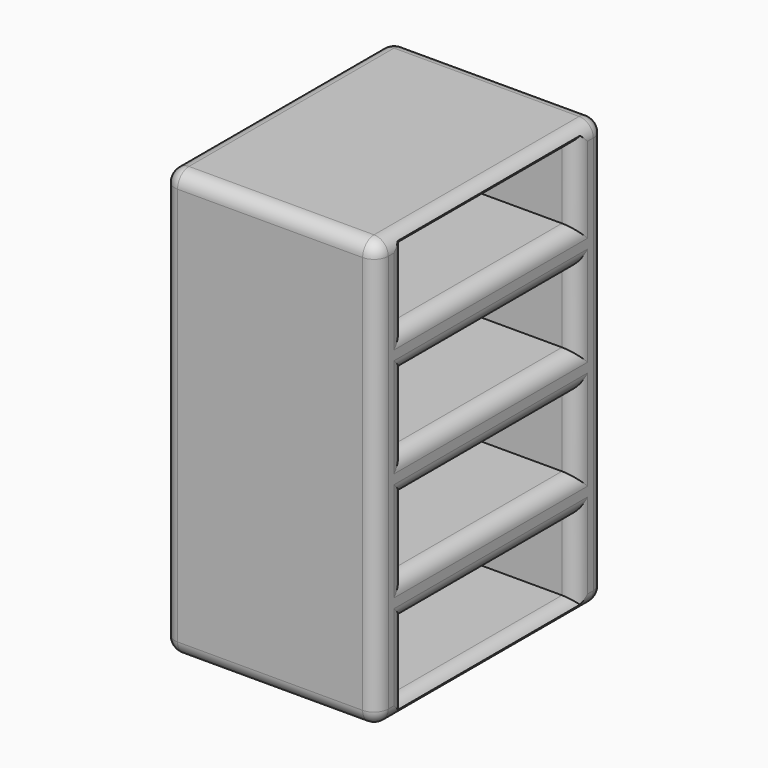
from build123d import *

# Parameters (mm, degrees)
F0_W          = 76.2
F0_H          = 101.6
F1_DEPTH      = 152.4
F2_W          = 76.2
F2_H          = 25.4
F3_DEPTH      = 63.5
F4_T1_DEPTH   = 101.6
F4_T3_DEPTH   = 38.1
F4_T5_DEPTH   = 50.8
F4_T7_DEPTH   = 50.8
F4_T9_DEPTH   = 38.1
F4_T11_DEPTH  = 142.24
F4_T13_DEPTH  = 66.04
F4_T15_DEPTH  = 91.44
F4_T17_DEPTH  = 25.4
F4_T19_DEPTH  = 76.2
F4_T21_DEPTH  = 25.4
F4_T23_DEPTH  = 25.4
F4_T25_DEPTH  = 25.4
F4_S29_W      = 5.1816
F4_S29_H      = 5.1816
F4_T30_DEPTH  = 5.1816
F4_S35_W      = 5.1816
F4_S35_H      = 5.1816
F4_T36_DEPTH  = 5.1816
F4_S41_W      = 5.1816
F4_S41_H      = 5.1816
F4_T42_DEPTH  = 5.1816
F4_S47_W      = 5.1816
F4_S47_H      = 5.1816
F4_T48_DEPTH  = 5.1816
F4_S53_W      = 5.1816
F4_S53_H      = 5.1816
F4_T54_DEPTH  = 5.1816
F4_S59_W      = 5.1816
F4_S59_H      = 5.1816
F4_T60_DEPTH  = 5.1816
F4_S65_W      = 5.1816
F4_S65_H      = 5.1816
F4_T66_DEPTH  = 5.1816
F4_S71_W      = 5.1816
F4_S71_H      = 5.1816
F4_T72_DEPTH  = 5.1816
F4_T79_DEPTH  = 38.1
F4_T84_DEPTH  = 88.9
F4_T91_DEPTH  = 38.1
F4_T95_DEPTH  = 88.9
F4_T102_DEPTH = 88.9
F4_T106_DEPTH = 38.1
F4_T114_DEPTH = 38.1
F4_T118_DEPTH = 88.9
F4_T125_DEPTH = 38.1
F4_T129_DEPTH = 88.9
F4_T136_DEPTH = 38.1
F4_T140_DEPTH = 88.9
F4_T147_DEPTH = 88.9
F4_T151_DEPTH = 38.1
F4_T158_DEPTH = 38.1
F4_T162_DEPTH = 88.9
F4_T169_DEPTH = 38.1
F4_T173_DEPTH = 88.9
F4_T180_DEPTH = 38.1
F4_T184_DEPTH = 88.9
F4_T191_DEPTH = 88.9
F4_T195_DEPTH = 38.1
F4_T202_DEPTH = 38.1
F4_T206_DEPTH = 88.9
F4_T213_DEPTH = 38.1
F4_T217_DEPTH = 88.9
F4_T224_DEPTH = 38.1
F4_T229_DEPTH = 88.9
F4_T236_DEPTH = 88.9
F4_T240_DEPTH = 38.1
F4_T247_DEPTH = 38.1
F4_T252_DEPTH = 88.9


# Not quite as in the source:
# - a fillet or chamfer that OpenCascade refuses, or shapes differently, is made with other operations: its cross-section is extruded or revolved along the edge and cut away or added


with BuildPart() as f1:
    # F0 (on Top) → F1 (new body)
    with BuildSketch(Plane.XY):
        with Locations((2.9496792704, 19.608187279)):
            Rectangle(F0_W, F0_H)
    extrude(amount=F1_DEPTH)

    # F2 (on face) → F3 (cut)
    with BuildSketch(Plane.YZ.offset(41.0496792704)):
        with Locations((19.608187279, 134.62)):
            Rectangle(F2_W, F2_H)
        with Locations((19.608187279, 95.6733333333)):
            Rectangle(F2_W, F2_H)
        with Locations((19.608187279, 56.7266666667)):
            Rectangle(F2_W, F2_H)
        with Locations((19.608187279, 17.78)):
            Rectangle(F2_W, F2_H)
    extrude(amount=-F3_DEPTH, mode=Mode.SUBTRACT)

    # F4: fillet of radius 5.08 on 44 edges, made by hand

    # F4_s2 → F4_t1 (join)
    with BuildSketch(Plane.XZ.offset(-70.408187279)):
        with BuildLine():
            ThreePointArc((-17.3703207296, 121.92), (-20.962423178, 123.4078975516), (-22.4503207296, 127))
            Line((-22.4503207296, 127), (-22.4503207296, 121.92))
            Line((-22.4503207296, 121.92), (-17.3703207296, 121.92))
        make_face()
        with BuildLine():
            ThreePointArc((-17.3703207296, 147.32), (-20.962423178, 145.8321024484), (-22.4503207296, 142.24))
            Line((-22.4503207296, 142.24), (-22.4503207296, 147.32))
            Line((-22.4503207296, 147.32), (-17.3703207296, 147.32))
        make_face()
        with BuildLine():
            ThreePointArc((-17.3703207296, 82.9733333333), (-20.962423178, 84.4612308849), (-22.4503207296, 88.0533333333))
            Line((-22.4503207296, 88.0533333333), (-22.4503207296, 82.9733333333))
            Line((-22.4503207296, 82.9733333333), (-17.3703207296, 82.9733333333))
        make_face()
        with BuildLine():
            ThreePointArc((-17.3703207296, 108.3733333333), (-20.962423178, 106.8854357818), (-22.4503207296, 103.2933333333))
            Line((-22.4503207296, 103.2933333333), (-22.4503207296, 108.3733333333))
            Line((-22.4503207296, 108.3733333333), (-17.3703207296, 108.3733333333))
        make_face()
        with BuildLine():
            ThreePointArc((-17.3703207296, 44.0266666667), (-20.962423178, 45.5145642182), (-22.4503207296, 49.1066666667))
            Line((-22.4503207296, 49.1066666667), (-22.4503207296, 44.0266666667))
            Line((-22.4503207296, 44.0266666667), (-17.3703207296, 44.0266666667))
        make_face()
        with BuildLine():
            ThreePointArc((-17.3703207296, 69.4266666667), (-20.962423178, 67.9387691151), (-22.4503207296, 64.3466666667))
            Line((-22.4503207296, 64.3466666667), (-22.4503207296, 69.4266666667))
            Line((-22.4503207296, 69.4266666667), (-17.3703207296, 69.4266666667))
        make_face()
        with BuildLine():
            ThreePointArc((-17.3703207296, 5.08), (-20.962423178, 6.5678975516), (-22.4503207296, 10.16))
            Line((-22.4503207296, 10.16), (-22.4503207296, 5.08))
            Line((-22.4503207296, 5.08), (-17.3703207296, 5.08))
        make_face()
        with BuildLine():
            ThreePointArc((-17.3703207296, 30.48), (-20.962423178, 28.9921024484), (-22.4503207296, 25.4))
            Line((-22.4503207296, 25.4), (-22.4503207296, 30.48))
            Line((-22.4503207296, 30.48), (-17.3703207296, 30.48))
        make_face()
    extrude(amount=F4_T1_DEPTH)

    # F4_s4 → F4_t3 (join)
    with BuildSketch(Plane.XY.offset(109.22)):
        with BuildLine():
            ThreePointArc((-17.3703207296, 57.708187279), (-20.962423178, 56.2202897274), (-22.4503207296, 52.628187279))
            Line((-22.4503207296, 52.628187279), (-22.4503207296, 57.708187279))
            Line((-22.4503207296, 57.708187279), (-17.3703207296, 57.708187279))
        make_face()
        with BuildLine():
            ThreePointArc((-17.3703207296, -18.491812721), (-20.962423178, -17.0039151694), (-22.4503207296, -13.411812721))
            Line((-22.4503207296, -13.411812721), (-22.4503207296, -18.491812721))
            Line((-22.4503207296, -18.491812721), (-17.3703207296, -18.491812721))
        make_face()
    extrude(amount=F4_T3_DEPTH)

    # F4_s6 → F4_t5 (join)
    with BuildSketch(Plane.XY.offset(70.2733333333)):
        with BuildLine():
            ThreePointArc((-17.3703207296, 57.708187279), (-20.962423178, 56.2202897274), (-22.4503207296, 52.628187279))
            Line((-22.4503207296, 52.628187279), (-22.4503207296, 57.708187279))
            Line((-22.4503207296, 57.708187279), (-17.3703207296, 57.708187279))
        make_face()
        with BuildLine():
            ThreePointArc((-17.3703207296, -18.491812721), (-20.962423178, -17.0039151694), (-22.4503207296, -13.411812721))
            Line((-22.4503207296, -13.411812721), (-22.4503207296, -18.491812721))
            Line((-22.4503207296, -18.491812721), (-17.3703207296, -18.491812721))
        make_face()
    extrude(amount=F4_T5_DEPTH)

    # F4_s8 → F4_t7 (join)
    with BuildSketch(Plane.XY.offset(31.3266666667)):
        with BuildLine():
            ThreePointArc((-17.3703207296, 57.708187279), (-20.962423178, 56.2202897274), (-22.4503207296, 52.628187279))
            Line((-22.4503207296, 52.628187279), (-22.4503207296, 57.708187279))
            Line((-22.4503207296, 57.708187279), (-17.3703207296, 57.708187279))
        make_face()
        with BuildLine():
            ThreePointArc((-17.3703207296, -18.491812721), (-20.962423178, -17.0039151694), (-22.4503207296, -13.411812721))
            Line((-22.4503207296, -13.411812721), (-22.4503207296, -18.491812721))
            Line((-22.4503207296, -18.491812721), (-17.3703207296, -18.491812721))
        make_face()
    extrude(amount=F4_T7_DEPTH)

    # F4_s10 → F4_t9 (join)
    with BuildSketch(Plane.XY.offset(5.08)):
        with BuildLine():
            ThreePointArc((-17.3703207296, 57.708187279), (-20.962423178, 56.2202897274), (-22.4503207296, 52.628187279))
            Line((-22.4503207296, 52.628187279), (-22.4503207296, 57.708187279))
            Line((-22.4503207296, 57.708187279), (-17.3703207296, 57.708187279))
        make_face()
        with BuildLine():
            ThreePointArc((-17.3703207296, -18.491812721), (-20.962423178, -17.0039151694), (-22.4503207296, -13.411812721))
            Line((-22.4503207296, -13.411812721), (-22.4503207296, -18.491812721))
            Line((-22.4503207296, -18.491812721), (-17.3703207296, -18.491812721))
        make_face()
    extrude(amount=F4_T9_DEPTH)

    # F4_s12 → F4_t11 (cut)
    with BuildSketch(Plane.XY.offset(5.08)):
        with BuildLine():
            ThreePointArc((-35.1503207296, -26.111812721), (-33.662423178, -29.7039151694), (-30.0703207296, -31.191812721))
            Line((-30.0703207296, -31.191812721), (-35.1503207296, -31.191812721))
            Line((-35.1503207296, -31.191812721), (-35.1503207296, -26.111812721))
        make_face()
        with BuildLine():
            ThreePointArc((41.0496792704, -26.111812721), (39.5617817188, -29.7039151694), (35.9696792704, -31.191812721))
            Line((35.9696792704, -31.191812721), (41.0496792704, -31.191812721))
            Line((41.0496792704, -31.191812721), (41.0496792704, -26.111812721))
        make_face()
        with BuildLine():
            ThreePointArc((35.9696792704, 70.408187279), (39.5617817188, 68.9202897274), (41.0496792704, 65.328187279))
            Line((41.0496792704, 65.328187279), (41.0496792704, 70.408187279))
            Line((41.0496792704, 70.408187279), (35.9696792704, 70.408187279))
        make_face()
        with BuildLine():
            ThreePointArc((-30.0703207296, 70.408187279), (-33.662423178, 68.9202897274), (-35.1503207296, 65.328187279))
            Line((-35.1503207296, 65.328187279), (-35.1503207296, 70.408187279))
            Line((-35.1503207296, 70.408187279), (-30.0703207296, 70.408187279))
        make_face()
    extrude(amount=F4_T11_DEPTH, mode=Mode.SUBTRACT)

    # F4_s14 → F4_t13 (cut)
    with BuildSketch(Plane.YZ.offset(-30.0703207296)):
        with BuildLine():
            ThreePointArc((-26.111812721, 0), (-29.7039151694, 1.4878975516), (-31.191812721, 5.08))
            Line((-31.191812721, 5.08), (-31.191812721, 0))
            Line((-31.191812721, 0), (-26.111812721, 0))
        make_face()
        with BuildLine():
            ThreePointArc((-26.111812721, 152.4), (-29.7039151694, 150.9121024484), (-31.191812721, 147.32))
            Line((-31.191812721, 147.32), (-31.191812721, 152.4))
            Line((-31.191812721, 152.4), (-26.111812721, 152.4))
        make_face()
        with BuildLine():
            ThreePointArc((70.408187279, 5.08), (68.9202897274, 1.4878975516), (65.328187279, 0))
            Line((65.328187279, 0), (70.408187279, 0))
            Line((70.408187279, 0), (70.408187279, 5.08))
        make_face()
        with BuildLine():
            ThreePointArc((70.408187279, 147.32), (68.9202897274, 150.9121024484), (65.328187279, 152.4))
            Line((65.328187279, 152.4), (70.408187279, 152.4))
            Line((70.408187279, 152.4), (70.408187279, 147.32))
        make_face()
    extrude(amount=F4_T13_DEPTH, mode=Mode.SUBTRACT)

    # F4_s16 → F4_t15 (cut)
    with BuildSketch(Plane.XZ.offset(-65.328187279)):
        with BuildLine():
            ThreePointArc((-30.0703207296, 0), (-33.662423178, 1.4878975516), (-35.1503207296, 5.08))
            Line((-35.1503207296, 5.08), (-35.1503207296, 0))
            Line((-35.1503207296, 0), (-30.0703207296, 0))
        make_face()
        with BuildLine():
            ThreePointArc((41.0496792704, 5.08), (39.5617817188, 1.4878975516), (35.9696792704, 0))
            Line((35.9696792704, 0), (41.0496792704, 0))
            Line((41.0496792704, 0), (41.0496792704, 5.08))
        make_face()
        with BuildLine():
            ThreePointArc((-30.0703207296, 152.4), (-33.662423178, 150.9121024484), (-35.1503207296, 147.32))
            Line((-35.1503207296, 147.32), (-35.1503207296, 152.4))
            Line((-35.1503207296, 152.4), (-30.0703207296, 152.4))
        make_face()
        with BuildLine():
            ThreePointArc((41.0496792704, 147.32), (39.5617817188, 150.9121024484), (35.9696792704, 152.4))
            Line((35.9696792704, 152.4), (41.0496792704, 152.4))
            Line((41.0496792704, 152.4), (41.0496792704, 147.32))
        make_face()
    extrude(amount=F4_T15_DEPTH, mode=Mode.SUBTRACT)

    # F4_s18 → F4_t17 (cut)
    with BuildSketch(Plane.XY.offset(121.92)):
        with BuildLine():
            ThreePointArc((41.0496792704, -23.571812721), (39.5617817188, -19.9797102726), (35.9696792704, -18.491812721))
            Line((35.9696792704, -18.491812721), (41.0496792704, -18.491812721))
            Line((41.0496792704, -18.491812721), (41.0496792704, -23.571812721))
        make_face()
        with BuildLine():
            ThreePointArc((41.0496792704, 62.788187279), (39.5617817188, 59.1960848306), (35.9696792704, 57.708187279))
            Line((35.9696792704, 57.708187279), (41.0496792704, 57.708187279))
            Line((41.0496792704, 57.708187279), (41.0496792704, 62.788187279))
        make_face()
    extrude(amount=F4_T17_DEPTH, mode=Mode.SUBTRACT)

    # F4_s20 → F4_t19 (cut)
    with BuildSketch(Plane.XZ.offset(-57.708187279)):
        with BuildLine():
            ThreePointArc((41.0496792704, 152.4), (39.5617817188, 148.8078975516), (35.9696792704, 147.32))
            Line((35.9696792704, 147.32), (41.0496792704, 147.32))
            Line((41.0496792704, 147.32), (41.0496792704, 152.4))
        make_face()
        with BuildLine():
            ThreePointArc((41.0496792704, 116.84), (39.5617817188, 120.4321024484), (35.9696792704, 121.92))
            Line((35.9696792704, 121.92), (41.0496792704, 121.92))
            Line((41.0496792704, 121.92), (41.0496792704, 116.84))
        make_face()
        with BuildLine():
            ThreePointArc((41.0496792704, 113.4533333333), (39.5617817188, 109.8612308849), (35.9696792704, 108.3733333333))
            Line((35.9696792704, 108.3733333333), (41.0496792704, 108.3733333333))
            Line((41.0496792704, 108.3733333333), (41.0496792704, 113.4533333333))
        make_face()
        with BuildLine():
            ThreePointArc((41.0496792704, 77.8933333333), (39.5617817188, 81.4854357818), (35.9696792704, 82.9733333333))
            Line((35.9696792704, 82.9733333333), (41.0496792704, 82.9733333333))
            Line((41.0496792704, 82.9733333333), (41.0496792704, 77.8933333333))
        make_face()
        with BuildLine():
            ThreePointArc((41.0496792704, 74.5066666667), (39.5617817188, 70.9145642182), (35.9696792704, 69.4266666667))
            Line((35.9696792704, 69.4266666667), (41.0496792704, 69.4266666667))
            Line((41.0496792704, 69.4266666667), (41.0496792704, 74.5066666667))
        make_face()
        with BuildLine():
            ThreePointArc((41.0496792704, 38.9466666667), (39.5617817188, 42.5387691151), (35.9696792704, 44.0266666667))
            Line((35.9696792704, 44.0266666667), (41.0496792704, 44.0266666667))
            Line((41.0496792704, 44.0266666667), (41.0496792704, 38.9466666667))
        make_face()
        with BuildLine():
            ThreePointArc((41.0496792704, 35.56), (39.5617817188, 31.9678975516), (35.9696792704, 30.48))
            Line((35.9696792704, 30.48), (41.0496792704, 30.48))
            Line((41.0496792704, 30.48), (41.0496792704, 35.56))
        make_face()
        with BuildLine():
            ThreePointArc((41.0496792704, 0), (39.5617817188, 3.5921024484), (35.9696792704, 5.08))
            Line((35.9696792704, 5.08), (41.0496792704, 5.08))
            Line((41.0496792704, 5.08), (41.0496792704, 0))
        make_face()
    extrude(amount=F4_T19_DEPTH, mode=Mode.SUBTRACT)

    # F4_s22 → F4_t21 (cut)
    with BuildSketch(Plane.XY.offset(82.9733333333)):
        with BuildLine():
            ThreePointArc((41.0496792704, -23.571812721), (39.5617817188, -19.9797102726), (35.9696792704, -18.491812721))
            Line((35.9696792704, -18.491812721), (41.0496792704, -18.491812721))
            Line((41.0496792704, -18.491812721), (41.0496792704, -23.571812721))
        make_face()
        with BuildLine():
            ThreePointArc((41.0496792704, 62.788187279), (39.5617817188, 59.1960848306), (35.9696792704, 57.708187279))
            Line((35.9696792704, 57.708187279), (41.0496792704, 57.708187279))
            Line((41.0496792704, 57.708187279), (41.0496792704, 62.788187279))
        make_face()
    extrude(amount=F4_T21_DEPTH, mode=Mode.SUBTRACT)

    # F4_s24 → F4_t23 (cut)
    with BuildSketch(Plane.XY.offset(44.0266666667)):
        with BuildLine():
            ThreePointArc((41.0496792704, -23.571812721), (39.5617817188, -19.9797102726), (35.9696792704, -18.491812721))
            Line((35.9696792704, -18.491812721), (41.0496792704, -18.491812721))
            Line((41.0496792704, -18.491812721), (41.0496792704, -23.571812721))
        make_face()
        with BuildLine():
            ThreePointArc((41.0496792704, 62.788187279), (39.5617817188, 59.1960848306), (35.9696792704, 57.708187279))
            Line((35.9696792704, 57.708187279), (41.0496792704, 57.708187279))
            Line((41.0496792704, 57.708187279), (41.0496792704, 62.788187279))
        make_face()
    extrude(amount=F4_T23_DEPTH, mode=Mode.SUBTRACT)

    # F4_s26 → F4_t25 (cut)
    with BuildSketch(Plane.XY.offset(5.08)):
        with BuildLine():
            ThreePointArc((41.0496792704, -23.571812721), (39.5617817188, -19.9797102726), (35.9696792704, -18.491812721))
            Line((35.9696792704, -18.491812721), (41.0496792704, -18.491812721))
            Line((41.0496792704, -18.491812721), (41.0496792704, -23.571812721))
        make_face()
        with BuildLine():
            ThreePointArc((41.0496792704, 62.788187279), (39.5617817188, 59.1960848306), (35.9696792704, 57.708187279))
            Line((35.9696792704, 57.708187279), (41.0496792704, 57.708187279))
            Line((41.0496792704, 57.708187279), (41.0496792704, 62.788187279))
        make_face()
    extrude(amount=F4_T25_DEPTH, mode=Mode.SUBTRACT)


with BuildPart() as f4_tool28:
    # F4_s29 → F4_t30 (new body)
    with BuildSketch(Plane.XY.offset(5.08)):
        with Locations((-32.6611207296, -28.702612721)):
            Rectangle(F4_S29_W, F4_S29_H)
    extrude(amount=-F4_T30_DEPTH)

    # F4_s31 → F4_t32 (revolve, cut)
    with BuildSketch(Plane(origin=(-30.0703207296, -26.111812721, 5.08), x_dir=(0.7071067812, 0.7071067812, 0), z_dir=(-0.7071067812, 0.7071067812, 0))):
        with BuildLine():
            ThreePointArc((0, -5.08), (5.08, 0), (0, 5.08))
            Line((0, 5.08), (0, -5.08))
        make_face()
    revolve(axis=Axis((-30.0703207296, -26.111812721, 5.08), (0, 0, -1)), mode=Mode.SUBTRACT)


with BuildPart() as f1_1:
    add(f1.part)

    # F4_t27: cut F4_tool28
    add(f4_tool28.part, mode=Mode.SUBTRACT)


with BuildPart() as f4_tool34:
    # F4_s35 → F4_t36 (new body)
    with BuildSketch(Plane.XY.offset(147.32)):
        with Locations((-32.6611207296, -28.702612721)):
            Rectangle(F4_S35_W, F4_S35_H)
    extrude(amount=F4_T36_DEPTH)

    # F4_s37 → F4_t38 (revolve, cut)
    with BuildSketch(Plane(origin=(-30.0703207296, -26.111812721, 147.32), x_dir=(0.7071067812, 0.7071067812, 0), z_dir=(0.7071067812, -0.7071067812, 0))):
        with BuildLine():
            ThreePointArc((0, -5.08), (5.08, 0), (0, 5.08))
            Line((0, 5.08), (0, -5.08))
        make_face()
    revolve(axis=Axis((-30.0703207296, -26.111812721, 147.32), (0, 0, 1)), mode=Mode.SUBTRACT)


with BuildPart() as f1_2:
    add(f1_1.part)

    # F4_t33: cut F4_tool34
    add(f4_tool34.part, mode=Mode.SUBTRACT)


with BuildPart() as f4_tool40:
    # F4_s41 → F4_t42 (new body)
    with BuildSketch(Plane.YZ.offset(35.9696792704)):
        with Locations((-28.702612721, 2.4892)):
            Rectangle(F4_S41_W, F4_S41_H)
    extrude(amount=F4_T42_DEPTH)

    # F4_s43 → F4_t44 (revolve, cut)
    with BuildSketch(Plane(origin=(35.9696792704, -26.111812721, 5.08), x_dir=(0, 0.7071067812, 0.7071067812), z_dir=(0, 0.7071067812, -0.7071067812))):
        with BuildLine():
            ThreePointArc((0, -5.08), (5.08, 0), (0, 5.08))
            Line((0, 5.08), (0, -5.08))
        make_face()
    revolve(axis=Axis((35.9696792704, -26.111812721, 5.08), (1, 0, 0)), mode=Mode.SUBTRACT)


with BuildPart() as f1_3:
    add(f1_2.part)

    # F4_t39: cut F4_tool40
    add(f4_tool40.part, mode=Mode.SUBTRACT)


with BuildPart() as f4_tool46:
    # F4_s47 → F4_t48 (new body)
    with BuildSketch(Plane.YZ.offset(35.9696792704)):
        with Locations((-28.702612721, 149.9108)):
            Rectangle(F4_S47_W, F4_S47_H)
    extrude(amount=F4_T48_DEPTH)

    # F4_s49 → F4_t50 (revolve, cut)
    with BuildSketch(Plane(origin=(35.9696792704, -26.111812721, 147.32), x_dir=(0, 0.7071067812, -0.7071067812), z_dir=(0, -0.7071067812, -0.7071067812))):
        with BuildLine():
            ThreePointArc((0, -5.08), (5.08, 0), (0, 5.08))
            Line((0, 5.08), (0, -5.08))
        make_face()
    revolve(axis=Axis((35.9696792704, -26.111812721, 147.32), (1, 0, 0)), mode=Mode.SUBTRACT)


with BuildPart() as f1_4:
    add(f1_3.part)

    # F4_t45: cut F4_tool46
    add(f4_tool46.part, mode=Mode.SUBTRACT)


with BuildPart() as f4_tool52:
    # F4_s53 → F4_t54 (new body)
    with BuildSketch(Plane.XZ.offset(-65.328187279)):
        with Locations((38.5604792704, 2.4892)):
            Rectangle(F4_S53_W, F4_S53_H)
    extrude(amount=-F4_T54_DEPTH)

    # F4_s55 → F4_t56 (revolve, cut)
    with BuildSketch(Plane(origin=(35.9696792704, 65.328187279, 5.08), x_dir=(-0.7071067812, 0, 0.7071067812), z_dir=(-0.7071067812, 0, -0.7071067812))):
        with BuildLine():
            ThreePointArc((0, -5.08), (5.08, 0), (0, 5.08))
            Line((0, 5.08), (0, -5.08))
        make_face()
    revolve(axis=Axis((35.9696792704, 65.328187279, 5.08), (0, 1, 0)), mode=Mode.SUBTRACT)


with BuildPart() as f1_5:
    add(f1_4.part)

    # F4_t51: cut F4_tool52
    add(f4_tool52.part, mode=Mode.SUBTRACT)


with BuildPart() as f4_tool58:
    # F4_s59 → F4_t60 (new body)
    with BuildSketch(Plane.XZ.offset(-65.328187279)):
        with Locations((38.5604792704, 149.9108)):
            Rectangle(F4_S59_W, F4_S59_H)
    extrude(amount=-F4_T60_DEPTH)

    # F4_s61 → F4_t62 (revolve, cut)
    with BuildSketch(Plane(origin=(35.9696792704, 65.328187279, 147.32), x_dir=(-0.7071067812, 0, -0.7071067812), z_dir=(0.7071067812, 0, -0.7071067812))):
        with BuildLine():
            ThreePointArc((0, -5.08), (5.08, 0), (0, 5.08))
            Line((0, 5.08), (0, -5.08))
        make_face()
    revolve(axis=Axis((35.9696792704, 65.328187279, 147.32), (0, 1, 0)), mode=Mode.SUBTRACT)


with BuildPart() as f1_6:
    add(f1_5.part)

    # F4_t57: cut F4_tool58
    add(f4_tool58.part, mode=Mode.SUBTRACT)


with BuildPart() as f4_tool64:
    # F4_s65 → F4_t66 (new body)
    with BuildSketch(Plane.XZ.offset(-65.328187279)):
        with Locations((-32.6611207296, 2.4892)):
            Rectangle(F4_S65_W, F4_S65_H)
    extrude(amount=-F4_T66_DEPTH)

    # F4_s67 → F4_t68 (revolve, cut)
    with BuildSketch(Plane(origin=(-30.0703207296, 65.328187279, 5.08), x_dir=(0.7071067812, 0, 0.7071067812), z_dir=(-0.7071067812, 0, 0.7071067812))):
        with BuildLine():
            ThreePointArc((0, -5.08), (5.08, 0), (0, 5.08))
            Line((0, 5.08), (0, -5.08))
        make_face()
    revolve(axis=Axis((-30.0703207296, 65.328187279, 5.08), (0, 1, 0)), mode=Mode.SUBTRACT)


with BuildPart() as f1_7:
    add(f1_6.part)

    # F4_t63: cut F4_tool64
    add(f4_tool64.part, mode=Mode.SUBTRACT)


with BuildPart() as f4_tool70:
    # F4_s71 → F4_t72 (new body)
    with BuildSketch(Plane.XZ.offset(-65.328187279)):
        with Locations((-32.6611207296, 149.9108)):
            Rectangle(F4_S71_W, F4_S71_H)
    extrude(amount=-F4_T72_DEPTH)

    # F4_s73 → F4_t74 (revolve, cut)
    with BuildSketch(Plane(origin=(-30.0703207296, 65.328187279, 147.32), x_dir=(0.7071067812, 0, -0.7071067812), z_dir=(0.7071067812, 0, 0.7071067812))):
        with BuildLine():
            ThreePointArc((0, -5.08), (5.08, 0), (0, 5.08))
            Line((0, 5.08), (0, -5.08))
        make_face()
    revolve(axis=Axis((-30.0703207296, 65.328187279, 147.32), (0, 1, 0)), mode=Mode.SUBTRACT)


with BuildPart() as f1_8:
    add(f1_7.part)

    # F4_t69: cut F4_tool70
    add(f4_tool70.part, mode=Mode.SUBTRACT)


with BuildPart() as f4_tool77:
    # F4_s78 → F4_t79 (new body)
    with BuildSketch(Plane.XY.offset(160.02)):
        with BuildLine():
            ThreePointArc((41.0496792704, -23.571812721), (39.5617817188, -19.9797102726), (35.9696792704, -18.491812721))
            Line((35.9696792704, -18.491812721), (41.0496792704, -18.491812721))
            Line((41.0496792704, -18.491812721), (41.0496792704, -23.571812721))
        make_face()
    extrude(amount=-F4_T79_DEPTH)

    split(bisect_by=Plane.XY.offset(152.4), keep=Keep.BOTTOM)

    split(bisect_by=Plane.XY.offset(147.32), keep=Keep.TOP)


with BuildPart() as f4_tool82:
    # F4_s83 → F4_t84 (new body)
    with BuildSketch(Plane.XZ.offset(-57.708187279)):
        with BuildLine():
            ThreePointArc((41.0496792704, 152.4), (39.5617817188, 148.8078975516), (35.9696792704, 147.32))
            Line((35.9696792704, 147.32), (41.0496792704, 147.32))
            Line((41.0496792704, 147.32), (41.0496792704, 152.4))
        make_face()
    extrude(amount=F4_T84_DEPTH)

    split(bisect_by=Plane.XZ.offset(18.491812721), keep=Keep.TOP)


with BuildPart() as f4_tool77_1:
    add(f4_tool77.part)

    # F4_t86: intersect F4_tool82
    add(f4_tool82.part, mode=Mode.INTERSECT)


with BuildPart() as f1_9:
    add(f1_8.part)

    # F4_t75: cut F4_tool77
    add(f4_tool77_1.part, mode=Mode.SUBTRACT)


with BuildPart() as f4_tool89:
    # F4_s90 → F4_t91 (new body)
    with BuildSketch(Plane.XY.offset(147.32)):
        with BuildLine():
            ThreePointArc((41.0496792704, -23.571812721), (39.5617817188, -19.9797102726), (35.9696792704, -18.491812721))
            Line((35.9696792704, -18.491812721), (41.0496792704, -18.491812721))
            Line((41.0496792704, -18.491812721), (41.0496792704, -23.571812721))
        make_face()
    extrude(amount=-F4_T91_DEPTH)

    split(bisect_by=Plane.XY.offset(121.92), keep=Keep.BOTTOM)


with BuildPart() as f4_tool93:
    # F4_s94 → F4_t95 (new body)
    with BuildSketch(Plane.XZ.offset(31.191812721)):
        with BuildLine():
            ThreePointArc((41.0496792704, 116.84), (39.5617817188, 120.4321024484), (35.9696792704, 121.92))
            Line((35.9696792704, 121.92), (41.0496792704, 121.92))
            Line((41.0496792704, 121.92), (41.0496792704, 116.84))
        make_face()
    extrude(amount=-F4_T95_DEPTH)

    split(bisect_by=Plane.XZ.offset(18.491812721), keep=Keep.TOP)


with BuildPart() as f4_tool89_1:
    add(f4_tool89.part)

    # F4_t97: intersect F4_tool93
    add(f4_tool93.part, mode=Mode.INTERSECT)


with BuildPart() as f1_10:
    add(f1_9.part)

    # F4_t87: cut F4_tool89
    add(f4_tool89_1.part, mode=Mode.SUBTRACT)


with BuildPart() as f4_tool100:
    # F4_s101 → F4_t102 (new body)
    with BuildSketch(Plane.XZ.offset(-70.408187279)):
        with BuildLine():
            ThreePointArc((41.0496792704, 152.4), (39.5617817188, 148.8078975516), (35.9696792704, 147.32))
            Line((35.9696792704, 147.32), (41.0496792704, 147.32))
            Line((41.0496792704, 147.32), (41.0496792704, 152.4))
        make_face()
    extrude(amount=F4_T102_DEPTH)

    split(bisect_by=Plane.XZ.offset(-57.708187279), keep=Keep.BOTTOM)


with BuildPart() as f4_tool104:
    # F4_s105 → F4_t106 (new body)
    with BuildSketch(Plane.XY.offset(121.92)):
        with BuildLine():
            ThreePointArc((41.0496792704, 62.788187279), (39.5617817188, 59.1960848306), (35.9696792704, 57.708187279))
            Line((35.9696792704, 57.708187279), (41.0496792704, 57.708187279))
            Line((41.0496792704, 57.708187279), (41.0496792704, 62.788187279))
        make_face()
    extrude(amount=F4_T106_DEPTH)

    split(bisect_by=Plane.XY.offset(152.4), keep=Keep.BOTTOM)

    split(bisect_by=Plane.XY.offset(147.32), keep=Keep.TOP)


with BuildPart() as f4_tool100_1:
    add(f4_tool100.part)

    # F4_t109: intersect F4_tool104
    add(f4_tool104.part, mode=Mode.INTERSECT)


with BuildPart() as f1_11:
    add(f1_10.part)

    # F4_t98: cut F4_tool100
    add(f4_tool100_1.part, mode=Mode.SUBTRACT)


with BuildPart() as f4_tool112:
    # F4_s113 → F4_t114 (new body)
    with BuildSketch(Plane.XY.offset(109.22)):
        with BuildLine():
            ThreePointArc((41.0496792704, 62.788187279), (39.5617817188, 59.1960848306), (35.9696792704, 57.708187279))
            Line((35.9696792704, 57.708187279), (41.0496792704, 57.708187279))
            Line((41.0496792704, 57.708187279), (41.0496792704, 62.788187279))
        make_face()
    extrude(amount=F4_T114_DEPTH)

    split(bisect_by=Plane.XY.offset(121.92), keep=Keep.BOTTOM)


with BuildPart() as f4_tool116:
    # F4_s117 → F4_t118 (new body)
    with BuildSketch(Plane.XZ.offset(18.491812721)):
        with BuildLine():
            ThreePointArc((41.0496792704, 116.84), (39.5617817188, 120.4321024484), (35.9696792704, 121.92))
            Line((35.9696792704, 121.92), (41.0496792704, 121.92))
            Line((41.0496792704, 121.92), (41.0496792704, 116.84))
        make_face()
    extrude(amount=-F4_T118_DEPTH)

    split(bisect_by=Plane.XZ.offset(-57.708187279), keep=Keep.BOTTOM)


with BuildPart() as f4_tool112_1:
    add(f4_tool112.part)

    # F4_t120: intersect F4_tool116
    add(f4_tool116.part, mode=Mode.INTERSECT)


with BuildPart() as f1_12:
    add(f1_11.part)

    # F4_t110: cut F4_tool112
    add(f4_tool112_1.part, mode=Mode.SUBTRACT)


with BuildPart() as f4_tool123:
    # F4_s124 → F4_t125 (new body)
    with BuildSketch(Plane.XY.offset(121.0733333333)):
        with BuildLine():
            ThreePointArc((41.0496792704, -23.571812721), (39.5617817188, -19.9797102726), (35.9696792704, -18.491812721))
            Line((35.9696792704, -18.491812721), (41.0496792704, -18.491812721))
            Line((41.0496792704, -18.491812721), (41.0496792704, -23.571812721))
        make_face()
    extrude(amount=-F4_T125_DEPTH)

    split(bisect_by=Plane.XY.offset(108.3733333333), keep=Keep.TOP)


with BuildPart() as f4_tool127:
    # F4_s128 → F4_t129 (new body)
    with BuildSketch(Plane.XZ.offset(-57.708187279)):
        with BuildLine():
            ThreePointArc((41.0496792704, 113.4533333333), (39.5617817188, 109.8612308849), (35.9696792704, 108.3733333333))
            Line((35.9696792704, 108.3733333333), (41.0496792704, 108.3733333333))
            Line((41.0496792704, 108.3733333333), (41.0496792704, 113.4533333333))
        make_face()
    extrude(amount=F4_T129_DEPTH)

    split(bisect_by=Plane.XZ.offset(18.491812721), keep=Keep.TOP)


with BuildPart() as f4_tool123_1:
    add(f4_tool123.part)

    # F4_t131: intersect F4_tool127
    add(f4_tool127.part, mode=Mode.INTERSECT)


with BuildPart() as f1_13:
    add(f1_12.part)

    # F4_t121: cut F4_tool123
    add(f4_tool123_1.part, mode=Mode.SUBTRACT)


with BuildPart() as f4_tool134:
    # F4_s135 → F4_t136 (new body)
    with BuildSketch(Plane.XY.offset(108.3733333333)):
        with BuildLine():
            ThreePointArc((41.0496792704, -23.571812721), (39.5617817188, -19.9797102726), (35.9696792704, -18.491812721))
            Line((35.9696792704, -18.491812721), (41.0496792704, -18.491812721))
            Line((41.0496792704, -18.491812721), (41.0496792704, -23.571812721))
        make_face()
    extrude(amount=-F4_T136_DEPTH)

    split(bisect_by=Plane.XY.offset(82.9733333333), keep=Keep.BOTTOM)


with BuildPart() as f4_tool138:
    # F4_s139 → F4_t140 (new body)
    with BuildSketch(Plane.XZ.offset(31.191812721)):
        with BuildLine():
            ThreePointArc((41.0496792704, 77.8933333333), (39.5617817188, 81.4854357818), (35.9696792704, 82.9733333333))
            Line((35.9696792704, 82.9733333333), (41.0496792704, 82.9733333333))
            Line((41.0496792704, 82.9733333333), (41.0496792704, 77.8933333333))
        make_face()
    extrude(amount=-F4_T140_DEPTH)

    split(bisect_by=Plane.XZ.offset(18.491812721), keep=Keep.TOP)


with BuildPart() as f4_tool134_1:
    add(f4_tool134.part)

    # F4_t142: intersect F4_tool138
    add(f4_tool138.part, mode=Mode.INTERSECT)


with BuildPart() as f1_14:
    add(f1_13.part)

    # F4_t132: cut F4_tool134
    add(f4_tool134_1.part, mode=Mode.SUBTRACT)


with BuildPart() as f4_tool145:
    # F4_s146 → F4_t147 (new body)
    with BuildSketch(Plane.XZ.offset(-70.408187279)):
        with BuildLine():
            ThreePointArc((41.0496792704, 113.4533333333), (39.5617817188, 109.8612308849), (35.9696792704, 108.3733333333))
            Line((35.9696792704, 108.3733333333), (41.0496792704, 108.3733333333))
            Line((41.0496792704, 108.3733333333), (41.0496792704, 113.4533333333))
        make_face()
    extrude(amount=F4_T147_DEPTH)

    split(bisect_by=Plane.XZ.offset(-57.708187279), keep=Keep.BOTTOM)


with BuildPart() as f4_tool149:
    # F4_s150 → F4_t151 (new body)
    with BuildSketch(Plane.XY.offset(82.9733333333)):
        with BuildLine():
            ThreePointArc((41.0496792704, 62.788187279), (39.5617817188, 59.1960848306), (35.9696792704, 57.708187279))
            Line((35.9696792704, 57.708187279), (41.0496792704, 57.708187279))
            Line((41.0496792704, 57.708187279), (41.0496792704, 62.788187279))
        make_face()
    extrude(amount=F4_T151_DEPTH)

    split(bisect_by=Plane.XY.offset(108.3733333333), keep=Keep.TOP)


with BuildPart() as f4_tool145_1:
    add(f4_tool145.part)

    # F4_t153: intersect F4_tool149
    add(f4_tool149.part, mode=Mode.INTERSECT)


with BuildPart() as f1_15:
    add(f1_14.part)

    # F4_t143: cut F4_tool145
    add(f4_tool145_1.part, mode=Mode.SUBTRACT)


with BuildPart() as f4_tool156:
    # F4_s157 → F4_t158 (new body)
    with BuildSketch(Plane.XY.offset(70.2733333333)):
        with BuildLine():
            ThreePointArc((41.0496792704, 62.788187279), (39.5617817188, 59.1960848306), (35.9696792704, 57.708187279))
            Line((35.9696792704, 57.708187279), (41.0496792704, 57.708187279))
            Line((41.0496792704, 57.708187279), (41.0496792704, 62.788187279))
        make_face()
    extrude(amount=F4_T158_DEPTH)

    split(bisect_by=Plane.XY.offset(82.9733333333), keep=Keep.BOTTOM)


with BuildPart() as f4_tool160:
    # F4_s161 → F4_t162 (new body)
    with BuildSketch(Plane.XZ.offset(18.491812721)):
        with BuildLine():
            ThreePointArc((41.0496792704, 77.8933333333), (39.5617817188, 81.4854357818), (35.9696792704, 82.9733333333))
            Line((35.9696792704, 82.9733333333), (41.0496792704, 82.9733333333))
            Line((41.0496792704, 82.9733333333), (41.0496792704, 77.8933333333))
        make_face()
    extrude(amount=-F4_T162_DEPTH)

    split(bisect_by=Plane.XZ.offset(-57.708187279), keep=Keep.BOTTOM)


with BuildPart() as f4_tool156_1:
    add(f4_tool156.part)

    # F4_t164: intersect F4_tool160
    add(f4_tool160.part, mode=Mode.INTERSECT)


with BuildPart() as f1_16:
    add(f1_15.part)

    # F4_t154: cut F4_tool156
    add(f4_tool156_1.part, mode=Mode.SUBTRACT)


with BuildPart() as f4_tool167:
    # F4_s168 → F4_t169 (new body)
    with BuildSketch(Plane.XY.offset(82.1266666667)):
        with BuildLine():
            ThreePointArc((41.0496792704, -23.571812721), (39.5617817188, -19.9797102726), (35.9696792704, -18.491812721))
            Line((35.9696792704, -18.491812721), (41.0496792704, -18.491812721))
            Line((41.0496792704, -18.491812721), (41.0496792704, -23.571812721))
        make_face()
    extrude(amount=-F4_T169_DEPTH)

    split(bisect_by=Plane.XY.offset(69.4266666667), keep=Keep.TOP)


with BuildPart() as f4_tool171:
    # F4_s172 → F4_t173 (new body)
    with BuildSketch(Plane.XZ.offset(-57.708187279)):
        with BuildLine():
            ThreePointArc((41.0496792704, 74.5066666667), (39.5617817188, 70.9145642182), (35.9696792704, 69.4266666667))
            Line((35.9696792704, 69.4266666667), (41.0496792704, 69.4266666667))
            Line((41.0496792704, 69.4266666667), (41.0496792704, 74.5066666667))
        make_face()
    extrude(amount=F4_T173_DEPTH)

    split(bisect_by=Plane.XZ.offset(18.491812721), keep=Keep.TOP)


with BuildPart() as f4_tool167_1:
    add(f4_tool167.part)

    # F4_t175: intersect F4_tool171
    add(f4_tool171.part, mode=Mode.INTERSECT)


with BuildPart() as f1_17:
    add(f1_16.part)

    # F4_t165: cut F4_tool167
    add(f4_tool167_1.part, mode=Mode.SUBTRACT)


with BuildPart() as f4_tool178:
    # F4_s179 → F4_t180 (new body)
    with BuildSketch(Plane.XY.offset(69.4266666667)):
        with BuildLine():
            ThreePointArc((41.0496792704, -23.571812721), (39.5617817188, -19.9797102726), (35.9696792704, -18.491812721))
            Line((35.9696792704, -18.491812721), (41.0496792704, -18.491812721))
            Line((41.0496792704, -18.491812721), (41.0496792704, -23.571812721))
        make_face()
    extrude(amount=-F4_T180_DEPTH)

    split(bisect_by=Plane.XY.offset(44.0266666667), keep=Keep.BOTTOM)


with BuildPart() as f4_tool182:
    # F4_s183 → F4_t184 (new body)
    with BuildSketch(Plane.XZ.offset(31.191812721)):
        with BuildLine():
            ThreePointArc((41.0496792704, 38.9466666667), (39.5617817188, 42.5387691151), (35.9696792704, 44.0266666667))
            Line((35.9696792704, 44.0266666667), (41.0496792704, 44.0266666667))
            Line((41.0496792704, 44.0266666667), (41.0496792704, 38.9466666667))
        make_face()
    extrude(amount=-F4_T184_DEPTH)

    split(bisect_by=Plane.XZ.offset(18.491812721), keep=Keep.TOP)


with BuildPart() as f4_tool178_1:
    add(f4_tool178.part)

    # F4_t186: intersect F4_tool182
    add(f4_tool182.part, mode=Mode.INTERSECT)


with BuildPart() as f1_18:
    add(f1_17.part)

    # F4_t176: cut F4_tool178
    add(f4_tool178_1.part, mode=Mode.SUBTRACT)


with BuildPart() as f4_tool189:
    # F4_s190 → F4_t191 (new body)
    with BuildSketch(Plane.XZ.offset(-70.408187279)):
        with BuildLine():
            ThreePointArc((41.0496792704, 74.5066666667), (39.5617817188, 70.9145642182), (35.9696792704, 69.4266666667))
            Line((35.9696792704, 69.4266666667), (41.0496792704, 69.4266666667))
            Line((41.0496792704, 69.4266666667), (41.0496792704, 74.5066666667))
        make_face()
    extrude(amount=F4_T191_DEPTH)

    split(bisect_by=Plane.XZ.offset(-57.708187279), keep=Keep.BOTTOM)


with BuildPart() as f4_tool193:
    # F4_s194 → F4_t195 (new body)
    with BuildSketch(Plane.XY.offset(44.0266666667)):
        with BuildLine():
            ThreePointArc((41.0496792704, 62.788187279), (39.5617817188, 59.1960848306), (35.9696792704, 57.708187279))
            Line((35.9696792704, 57.708187279), (41.0496792704, 57.708187279))
            Line((41.0496792704, 57.708187279), (41.0496792704, 62.788187279))
        make_face()
    extrude(amount=F4_T195_DEPTH)

    split(bisect_by=Plane.XY.offset(69.4266666667), keep=Keep.TOP)


with BuildPart() as f4_tool189_1:
    add(f4_tool189.part)

    # F4_t197: intersect F4_tool193
    add(f4_tool193.part, mode=Mode.INTERSECT)


with BuildPart() as f1_19:
    add(f1_18.part)

    # F4_t187: cut F4_tool189
    add(f4_tool189_1.part, mode=Mode.SUBTRACT)


with BuildPart() as f4_tool200:
    # F4_s201 → F4_t202 (new body)
    with BuildSketch(Plane.XY.offset(31.3266666667)):
        with BuildLine():
            ThreePointArc((41.0496792704, 62.788187279), (39.5617817188, 59.1960848306), (35.9696792704, 57.708187279))
            Line((35.9696792704, 57.708187279), (41.0496792704, 57.708187279))
            Line((41.0496792704, 57.708187279), (41.0496792704, 62.788187279))
        make_face()
    extrude(amount=F4_T202_DEPTH)

    split(bisect_by=Plane.XY.offset(44.0266666667), keep=Keep.BOTTOM)


with BuildPart() as f4_tool204:
    # F4_s205 → F4_t206 (new body)
    with BuildSketch(Plane.XZ.offset(18.491812721)):
        with BuildLine():
            ThreePointArc((41.0496792704, 38.9466666667), (39.5617817188, 42.5387691151), (35.9696792704, 44.0266666667))
            Line((35.9696792704, 44.0266666667), (41.0496792704, 44.0266666667))
            Line((41.0496792704, 44.0266666667), (41.0496792704, 38.9466666667))
        make_face()
    extrude(amount=-F4_T206_DEPTH)

    split(bisect_by=Plane.XZ.offset(-57.708187279), keep=Keep.BOTTOM)


with BuildPart() as f4_tool200_1:
    add(f4_tool200.part)

    # F4_t208: intersect F4_tool204
    add(f4_tool204.part, mode=Mode.INTERSECT)


with BuildPart() as f1_20:
    add(f1_19.part)

    # F4_t198: cut F4_tool200
    add(f4_tool200_1.part, mode=Mode.SUBTRACT)


with BuildPart() as f4_tool211:
    # F4_s212 → F4_t213 (new body)
    with BuildSketch(Plane.XY.offset(43.18)):
        with BuildLine():
            ThreePointArc((41.0496792704, -23.571812721), (39.5617817188, -19.9797102726), (35.9696792704, -18.491812721))
            Line((35.9696792704, -18.491812721), (41.0496792704, -18.491812721))
            Line((41.0496792704, -18.491812721), (41.0496792704, -23.571812721))
        make_face()
    extrude(amount=-F4_T213_DEPTH)

    split(bisect_by=Plane.XY.offset(30.48), keep=Keep.TOP)


with BuildPart() as f4_tool215:
    # F4_s216 → F4_t217 (new body)
    with BuildSketch(Plane.XZ.offset(-57.708187279)):
        with BuildLine():
            ThreePointArc((41.0496792704, 35.56), (39.5617817188, 31.9678975516), (35.9696792704, 30.48))
            Line((35.9696792704, 30.48), (41.0496792704, 30.48))
            Line((41.0496792704, 30.48), (41.0496792704, 35.56))
        make_face()
    extrude(amount=F4_T217_DEPTH)

    split(bisect_by=Plane.XZ.offset(18.491812721), keep=Keep.TOP)


with BuildPart() as f4_tool211_1:
    add(f4_tool211.part)

    # F4_t219: intersect F4_tool215
    add(f4_tool215.part, mode=Mode.INTERSECT)


with BuildPart() as f1_21:
    add(f1_20.part)

    # F4_t209: cut F4_tool211
    add(f4_tool211_1.part, mode=Mode.SUBTRACT)


with BuildPart() as f4_tool222:
    # F4_s223 → F4_t224 (new body)
    with BuildSketch(Plane.XY.offset(30.48)):
        with BuildLine():
            ThreePointArc((41.0496792704, -23.571812721), (39.5617817188, -19.9797102726), (35.9696792704, -18.491812721))
            Line((35.9696792704, -18.491812721), (41.0496792704, -18.491812721))
            Line((41.0496792704, -18.491812721), (41.0496792704, -23.571812721))
        make_face()
    extrude(amount=-F4_T224_DEPTH)

    split(bisect_by=Plane.XY, keep=Keep.TOP)

    split(bisect_by=Plane.XY.offset(5.08), keep=Keep.BOTTOM)


with BuildPart() as f4_tool227:
    # F4_s228 → F4_t229 (new body)
    with BuildSketch(Plane.XZ.offset(31.191812721)):
        with BuildLine():
            ThreePointArc((41.0496792704, 0), (39.5617817188, 3.5921024484), (35.9696792704, 5.08))
            Line((35.9696792704, 5.08), (41.0496792704, 5.08))
            Line((41.0496792704, 5.08), (41.0496792704, 0))
        make_face()
    extrude(amount=-F4_T229_DEPTH)

    split(bisect_by=Plane.XZ.offset(18.491812721), keep=Keep.TOP)


with BuildPart() as f4_tool222_1:
    add(f4_tool222.part)

    # F4_t231: intersect F4_tool227
    add(f4_tool227.part, mode=Mode.INTERSECT)


with BuildPart() as f1_22:
    add(f1_21.part)

    # F4_t220: cut F4_tool222
    add(f4_tool222_1.part, mode=Mode.SUBTRACT)


with BuildPart() as f4_tool234:
    # F4_s235 → F4_t236 (new body)
    with BuildSketch(Plane.XZ.offset(-70.408187279)):
        with BuildLine():
            ThreePointArc((41.0496792704, 35.56), (39.5617817188, 31.9678975516), (35.9696792704, 30.48))
            Line((35.9696792704, 30.48), (41.0496792704, 30.48))
            Line((41.0496792704, 30.48), (41.0496792704, 35.56))
        make_face()
    extrude(amount=F4_T236_DEPTH)

    split(bisect_by=Plane.XZ.offset(-57.708187279), keep=Keep.BOTTOM)


with BuildPart() as f4_tool238:
    # F4_s239 → F4_t240 (new body)
    with BuildSketch(Plane.XY.offset(5.08)):
        with BuildLine():
            ThreePointArc((41.0496792704, 62.788187279), (39.5617817188, 59.1960848306), (35.9696792704, 57.708187279))
            Line((35.9696792704, 57.708187279), (41.0496792704, 57.708187279))
            Line((41.0496792704, 57.708187279), (41.0496792704, 62.788187279))
        make_face()
    extrude(amount=F4_T240_DEPTH)

    split(bisect_by=Plane.XY.offset(30.48), keep=Keep.TOP)


with BuildPart() as f4_tool234_1:
    add(f4_tool234.part)

    # F4_t242: intersect F4_tool238
    add(f4_tool238.part, mode=Mode.INTERSECT)


with BuildPart() as f1_23:
    add(f1_22.part)

    # F4_t232: cut F4_tool234
    add(f4_tool234_1.part, mode=Mode.SUBTRACT)


with BuildPart() as f4_tool245:
    # F4_s246 → F4_t247 (new body)
    with BuildSketch(Plane.XY.offset(-7.62)):
        with BuildLine():
            ThreePointArc((41.0496792704, 62.788187279), (39.5617817188, 59.1960848306), (35.9696792704, 57.708187279))
            Line((35.9696792704, 57.708187279), (41.0496792704, 57.708187279))
            Line((41.0496792704, 57.708187279), (41.0496792704, 62.788187279))
        make_face()
    extrude(amount=F4_T247_DEPTH)

    split(bisect_by=Plane.XY, keep=Keep.TOP)

    split(bisect_by=Plane.XY.offset(5.08), keep=Keep.BOTTOM)


with BuildPart() as f4_tool250:
    # F4_s251 → F4_t252 (new body)
    with BuildSketch(Plane.XZ.offset(18.491812721)):
        with BuildLine():
            ThreePointArc((41.0496792704, 0), (39.5617817188, 3.5921024484), (35.9696792704, 5.08))
            Line((35.9696792704, 5.08), (41.0496792704, 5.08))
            Line((41.0496792704, 5.08), (41.0496792704, 0))
        make_face()
    extrude(amount=-F4_T252_DEPTH)

    split(bisect_by=Plane.XZ.offset(-57.708187279), keep=Keep.BOTTOM)


with BuildPart() as f4_tool245_1:
    add(f4_tool245.part)

    # F4_t254: intersect F4_tool250
    add(f4_tool250.part, mode=Mode.INTERSECT)


with BuildPart() as f1_24:
    add(f1_23.part)

    # F4_t243: cut F4_tool245
    add(f4_tool245_1.part, mode=Mode.SUBTRACT)


solid = f1_24.part
